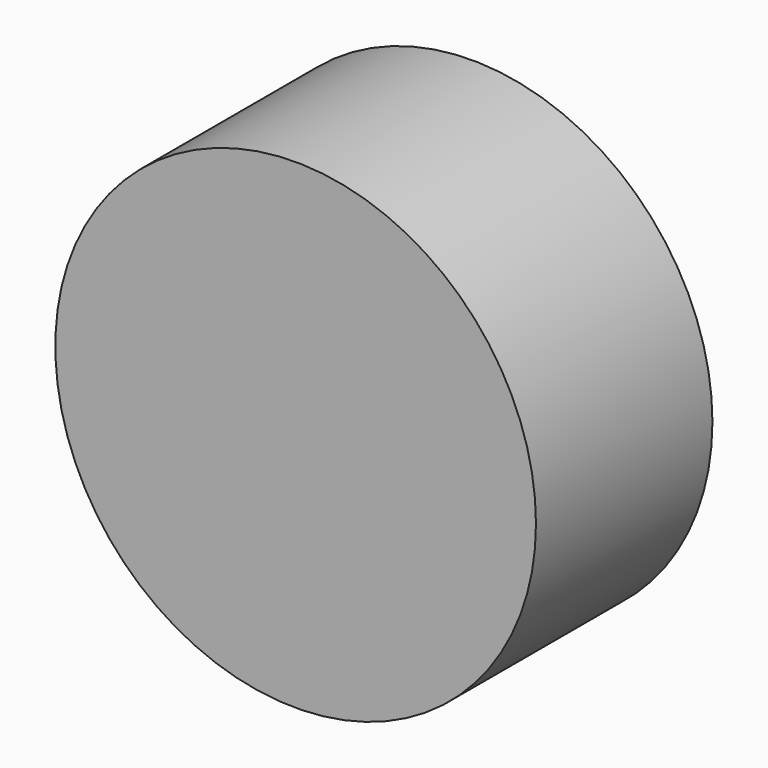
from build123d import *

# Parameters (mm, degrees)
F2_R     = 19.3718075752
F4_DEPTH = 8.89


# Not quite as in the source:
# - the program builds the solid bodies; features that only make, move or delete a surface that nothing else refers to are left out


with BuildPart() as f4:
    # F2 (on face) → F4 (new body, symmetric)
    with BuildSketch(Plane.XZ):
        Circle(F2_R)
    extrude(amount=F4_DEPTH, both=True)


solid = f4.part
